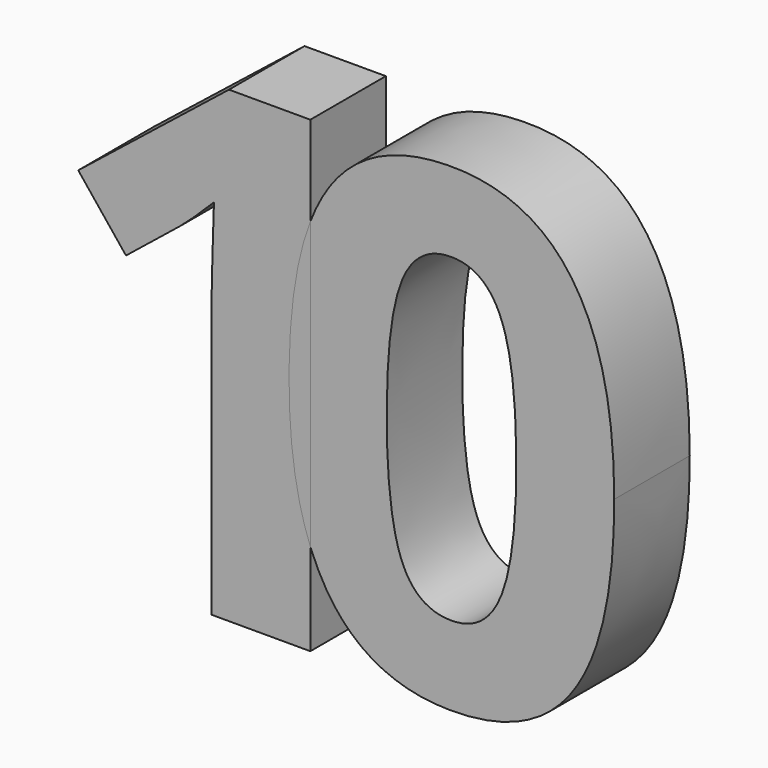
from build123d import *

# Parameters (mm, degrees)
F0_TEXT_SIZE = 13.8888888889
F1_DEPTH     = 2
F2_TEXT_SIZE = 13.8098205854
F3_DEPTH     = 2


# Not quite as in the source:
# - Text() gives the source's letters only with a copy of the font that has no kerning and outlines rounded to 1/6400 em; it was checked with that copy


with BuildPart() as f1:
    # F0 (on Front) → F1 (new body)
    with BuildSketch(Plane.XZ):
        with Locations((0, 0)):
            Text('1', F0_TEXT_SIZE, font='Open Sans', font_style=FontStyle.BOLD, text_align=(TextAlign.LEFT, TextAlign.BOTTOM))
    extrude(amount=F1_DEPTH)

    # F2 (on Front) → F3 (join)
    with BuildSketch(Plane.XZ):
        with Locations((4.7875165474, 0)):
            Text('0', F2_TEXT_SIZE, font='Open Sans', font_style=FontStyle.BOLD, text_align=(TextAlign.LEFT, TextAlign.BOTTOM))
    extrude(amount=F3_DEPTH)


solid = f1.part
